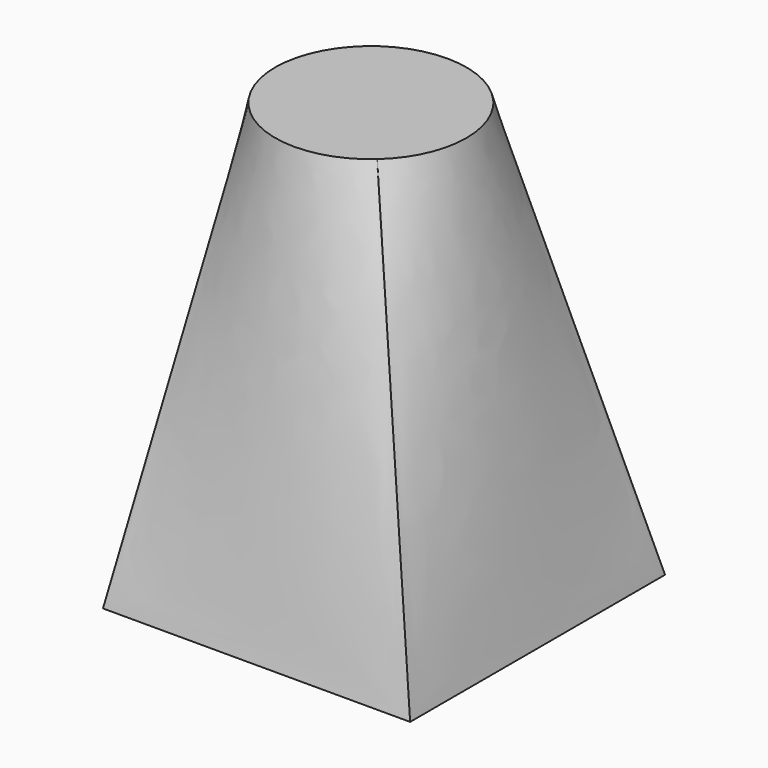
from build123d import *

# Parameters (mm, degrees)
F0_W = 55.9131167829
F0_H = 57.9994283617


# Not quite as in the source:
# - the arcs of a loft's sections are written as splines that run evenly, so that the points pair up as in the source's solid


with BuildPart() as f3:
    # F0 (on Top) → F3 section 0
    with BuildSketch(Plane.XY):
        with Locations((-2.0863097161, 2.190625295)):
            Rectangle(F0_W, F0_H)
    # F2 (on offset) → F3 section 1
    with BuildSketch(Plane.XY.offset(76.2)):
        with BuildLine():
            add(Edge.make_bspline(
                [(-17.692606509, 17.2795154284), (-18.5448195866, 16.5229064446), (-19.3224939536, 15.682382583), (-20.6989558576, 13.8657236269), (-21.2977093588, 12.8896334528), (-22.2933103526, 10.8393466931), (-22.6901332268, 9.7652008047), (-23.2666129225, 7.5600776116), (-23.4462554892, 6.429154833), (-23.5814600953, 4.1539368543), (-23.5370187915, 3.0096979135), (-23.2257524708, 0.7518205002), (-22.9589351508, -0.3617621419), (-22.2131596936, -2.5155300272), (-21.7342199972, -3.5556620142), (-20.5825951361, -5.5225522793), (-19.9099384474, -6.4492619222), (-19.1533294636, -7.3014749999)],
                knots=[0, 0, 0, 0, 0.125, 0.125, 0.25, 0.25, 0.375, 0.375, 0.5, 0.5, 0.625, 0.625, 0.75, 0.75, 0.875, 0.875, 1, 1, 1, 1], degree=3))
            add(Edge.make_bspline(
                [(-19.1533294636, -7.3014749999), (-18.3967204798, -8.1536880775), (-17.5561966182, -8.9313624445), (-15.7395376621, -10.3078243485), (-14.7634474881, -10.9065778497), (-12.7131607283, -11.9021788435), (-11.6390148399, -12.2990017177), (-9.4338916468, -12.8754814134), (-8.3029688682, -13.0551239801), (-6.0277508895, -13.1903285862), (-4.8835119487, -13.1458872824), (-2.6256345354, -12.8346209617), (-1.5120518933, -12.5678036417), (0.641715992, -11.8220281845), (1.681847979, -11.3430884881), (3.6487382441, -10.191463627), (4.575447887, -9.5188069383), (5.4276609647, -8.7621979545)],
                knots=[0, 0, 0, 0, 0.125, 0.125, 0.25, 0.25, 0.375, 0.375, 0.5, 0.5, 0.625, 0.625, 0.75, 0.75, 0.875, 0.875, 1, 1, 1, 1], degree=3))
            add(Edge.make_bspline(
                [(5.4276609647, -8.7621979545), (6.2798740423, -8.0055889707), (7.0575484093, -7.1650651091), (8.4340103133, -5.348406153), (9.0327638145, -4.372315979), (10.0283648083, -2.3220292192), (10.4251876825, -1.2478833308), (11.0016673782, 0.9572398623), (11.1813099449, 2.0881626409), (11.316514551, 4.3633806196), (11.2720732472, 5.5076195604), (10.9608069265, 7.7654969737), (10.6939896065, 8.8790796158), (9.9482141493, 11.0328475011), (9.4692744529, 12.072979488), (8.3176495918, 14.0398697532), (7.6449929031, 14.9665793961), (6.8883839193, 15.8187924737)],
                knots=[0, 0, 0, 0, 0.125, 0.125, 0.25, 0.25, 0.375, 0.375, 0.5, 0.5, 0.625, 0.625, 0.75, 0.75, 0.875, 0.875, 1, 1, 1, 1], degree=3))
            add(Edge.make_bspline(
                [(6.8883839193, 15.8187924737), (6.1317749355, 16.6710055514), (5.2912510739, 17.4486799184), (3.4745921178, 18.8251418224), (2.4985019438, 19.4238953236), (0.448215184, 20.4194963174), (-0.6259307044, 20.8163191916), (-2.8310538975, 21.3927988873), (-3.9619766761, 21.572441454), (-6.2371946548, 21.7076460601), (-7.3814335956, 21.6632047563), (-9.6393110089, 21.3519384356), (-10.752893651, 21.0851211156), (-12.9066615363, 20.3393456584), (-13.9467935233, 19.860405962), (-15.9136837884, 18.7087811009), (-16.8403934313, 18.0361244122), (-17.692606509, 17.2795154284)],
                knots=[0, 0, 0, 0, 0.125, 0.125, 0.25, 0.25, 0.375, 0.375, 0.5, 0.5, 0.625, 0.625, 0.75, 0.75, 0.875, 0.875, 1, 1, 1, 1], degree=3))
        make_face()
    loft(ruled=True)


solid = f3.part
